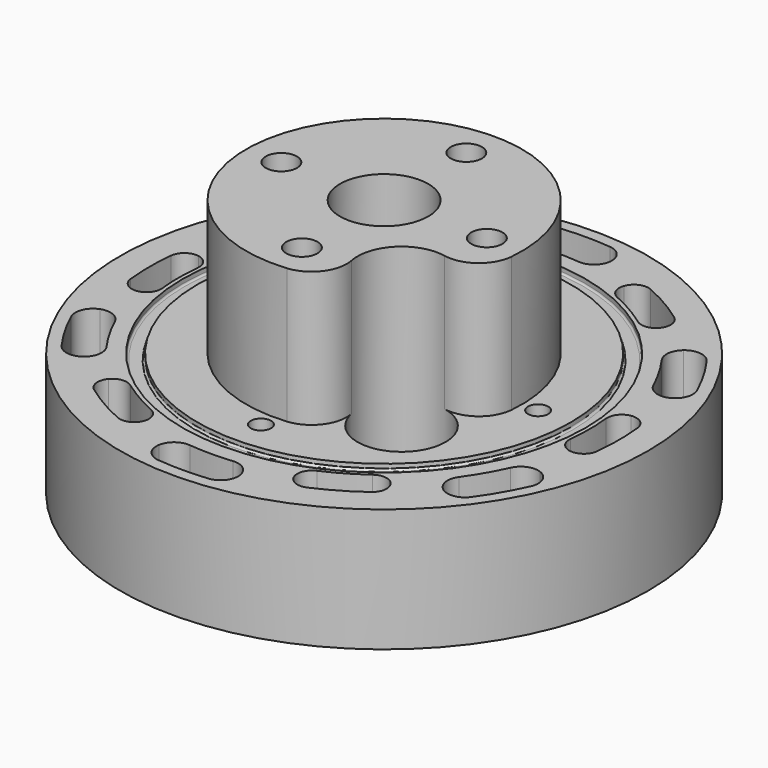
from build123d import *

# Parameters (mm, degrees)
F0_R             = 57.15
F1_DEPTH         = 19.05
F2_R             = 29.87
F2_R_2           = 9.55
F3_DEPTH         = 29.21
F5_D             = 6.7564
F6_R             = 57.15
F6_R_2           = 37.846
F7_DEPTH         = 7.62
F8_R             = 9.525
F9_DEPTH         = 55.881
F10_R            = 7.62
F11_R            = 43.6245
F11_R_2          = 40.4241
F12_DEPTH        = 1.2954
F13_R            = 0.4064
F15_DEPTH        = 26.671
F15_COPIES_COUNT = 6
F16_R            = 3.80999
F17_R            = 3.17499
F19_D            = 4.3942
F19_DEPTH        = 10.16
F19_TIP          = 1.3201508661


# Not quite as in the source:
# - a fillet or chamfer is up to 0.001 mm smaller than in the source, because OpenCascade refuses the exact size
# - a pattern or mirror of a feature is missing from the dataset's text; its kind, count and spacing are read off the source's solid


with BuildPart() as f1:
    # F0 (on Top) → F1 (new body)
    with BuildSketch(Plane.XY):
        Circle(F0_R)
    extrude(amount=F1_DEPTH)

    # F2 (on face) → F3 (join)
    with BuildSketch(Plane.XY.offset(19.05)):
        Circle(F2_R)
        Circle(F2_R_2, mode=Mode.SUBTRACT)
    extrude(amount=F3_DEPTH)

    # F5 (through all)
    with Locations(Plane.XY.offset(48.26)):
        with Locations((-22.25, 0), (0, 22.25), (22.25, 0), (0, -22.25)):
            Hole(F5_D / 2)

    # F6 (on face) → F7 (join)
    with BuildSketch(Plane(origin=(0, 0, 0), x_dir=(1, 0, 0), z_dir=(0, 0, -1))):
        Circle(F6_R)
        Circle(F6_R_2, mode=Mode.SUBTRACT)
    extrude(amount=F7_DEPTH)

    # F8 (on face) → F9 (cut, through all)
    with BuildSketch(Plane.XY.offset(48.26)):
        with Locations((18.8585378542, -18.8585378542)):
            Circle(F8_R)
    extrude(amount=-F9_DEPTH, mode=Mode.SUBTRACT)

    # F10
    f10_edges = [f1.edges().sort_by_distance(p)[0] for p in [
        (26.682506, -13.426122, 33.655),
        (13.426122, -26.682506, 33.655),
    ]]
    fillet(f10_edges, radius=F10_R)

    # F11 (on face) → F12 (cut)
    with BuildSketch(Plane.XY.offset(19.05)):
        Circle(F11_R)
        Circle(F11_R_2, mode=Mode.SUBTRACT)
    extrude(amount=-F12_DEPTH, mode=Mode.SUBTRACT)

    # F13
    f13_edges = [f1.edges().sort_by_distance(p)[0] for p in [
        (-40.4241, 0, 17.7546),
        (-43.6245, 0, 17.7546),
    ]]
    fillet(f13_edges, radius=F13_R)

    # F14 (on face) → F15 (cut, through all)
    with BuildSketch(Plane.XY.offset(19.05)):
        with BuildLine():
            ThreePointArc((-43.7747046214, -7.7186614973), (-44.45, 0), (-43.7747046214, 7.7186614973))
            Line((-43.7747046214, 7.7186614973), (-50.028233853, 8.8213274255))
            ThreePointArc((-50.028233853, 8.8213274255), (-50.8, 0), (-50.028233853, -8.8213274255))
            Line((-50.028233853, -8.8213274255), (-43.7747046214, -7.7186614973))
        make_face()
        with BuildLine():
            Line((-51.3166140211, 18.677720027), (-44.1561562507, 16.0715265349))
            ThreePointArc((-44.1561562507, 16.0715265349), (-40.6945337238, 23.495), (-35.9964283822, 30.2045897792))
            Line((-35.9964283822, 30.2045897792), (-41.8336870387, 35.102631365))
            ThreePointArc((-41.8336870387, 35.102631365), (-47.2936473007, 27.305), (-51.3166140211, 18.677720027))
        make_face()
    f15 = extrude(amount=-F15_DEPTH, mode=Mode.SUBTRACT)

    # F15_copies: F15 ×6 about axis
    f15_copies_axis = Axis((0, 0, 0), (0, 0, 1))
    for i in range(1, F15_COPIES_COUNT):
        add(f15.rotate(f15_copies_axis, i * 360 / F15_COPIES_COUNT), mode=Mode.SUBTRACT)

    # F16 (radius 3.81 in the source; OpenCascade refuses exactly that, so slightly less here)
    f16_edges = [f1.edges().sort_by_distance(p)[0] for p in [
        (-41.833687, 35.102631, 5.715),
        (-35.996428, 30.20459, 5.715),
        (-44.156156, 16.071527, 5.715),
        (-51.316614, 18.67772, 5.715),
        (-51.316614, -18.67772, 5.715),
        (-44.156156, -16.071527, 5.715),
        (-35.996428, -30.20459, 5.715),
        (-41.833687, -35.102631, 5.715),
        (-9.482927, -53.780351, 5.715),
        (-8.159728, -46.276116, 5.715),
        (8.159728, -46.276116, 5.715),
        (9.482927, -53.780351, 5.715),
        (41.833687, -35.102631, 5.715),
        (35.996428, -30.20459, 5.715),
        (44.156156, -16.071527, 5.715),
        (51.316614, -18.67772, 5.715),
        (9.482927, 53.780351, 5.715),
        (8.159728, 46.276116, 5.715),
        (-9.482927, 53.780351, 5.715),
        (-8.159728, 46.276116, 5.715),
        (51.316614, 18.67772, 5.715),
        (44.156156, 16.071527, 5.715),
        (35.996428, 30.20459, 5.715),
        (41.833687, 35.102631, 5.715),
    ]]
    fillet(f16_edges, radius=F16_R)

    # F17 (radius 3.175 in the source; OpenCascade refuses exactly that, so slightly less here)
    f17_edges = [f1.edges().sort_by_distance(p)[0] for p in [
        (-43.774705, 7.718661, 5.715),
        (-50.028234, 8.821327, 5.715),
        (-43.774705, -7.718661, 5.715),
        (-50.028234, -8.821327, 5.715),
        (-17.374623, -47.736385, 5.715),
        (-32.653611, -38.915058, 5.715),
        (-28.571909, -34.050675, 5.715),
        (-15.202795, -41.769337, 5.715),
        (32.653611, -38.915058, 5.715),
        (17.374623, -47.736385, 5.715),
        (15.202795, -41.769337, 5.715),
        (28.571909, -34.050675, 5.715),
        (-32.653611, 38.915058, 5.715),
        (-17.374623, 47.736385, 5.715),
        (-28.571909, 34.050675, 5.715),
        (-15.202795, 41.769337, 5.715),
        (50.028234, 8.821327, 5.715),
        (50.028234, -8.821327, 5.715),
        (43.774705, -7.718661, 5.715),
        (43.774705, 7.718661, 5.715),
        (17.374623, 47.736385, 5.715),
        (32.653611, 38.915058, 5.715),
        (28.571909, 34.050675, 5.715),
        (15.202795, 41.769337, 5.715),
    ]]
    fillet(f17_edges, radius=F17_R)

    # F19
    with Locations(Plane.XY.offset(19.05)):
        with Locations((33.3375, 0), (0, -33.3375), (-33.3375, 0), (0, 33.3375)):
            Hole(F19_D / 2, depth=F19_DEPTH)
            with Locations((0, 0, -(F19_DEPTH + F19_TIP / 2))):  # 118° drill point
                Cone(0, F19_D / 2, F19_TIP, mode=Mode.SUBTRACT)


solid = f1.part
